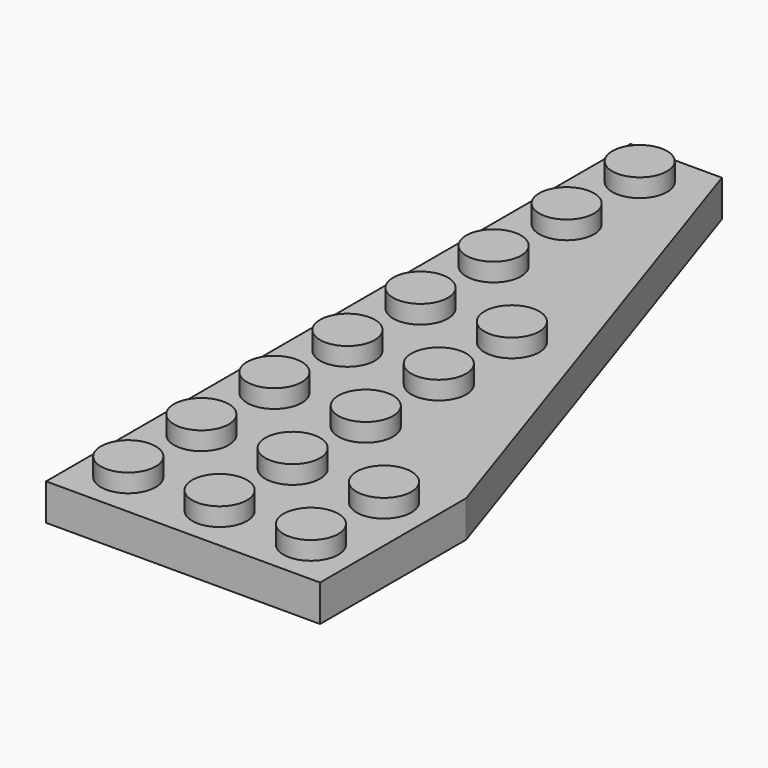
from build123d import *

# Parameters (mm, degrees)
F0_R     = 2.38125
F1_DEPTH = 3.175
F2_DEPTH = 4.7625
F3_T     = -1.5875
F4_R     = 3.175
F4_R_2   = 2.38125
F5_DEPTH = 1.5875


with BuildPart() as f1:
    # F0 (on Top) → F1 (new body)
    with BuildSketch(Plane.XY):
        Polygon((-3.96875, 31.75), (-11.90625, 31.75), (-11.90625, -31.75), (11.90625, -31.75), (11.90625, -15.875), align=None)
        with Locations((-7.9375, -27.78125)):
            Circle(F0_R, mode=Mode.SUBTRACT)
        with Locations((-7.9375, -19.84375)):
            Circle(F0_R, mode=Mode.SUBTRACT)
        with Locations((-7.9375, -11.90625)):
            Circle(F0_R, mode=Mode.SUBTRACT)
        with Locations((-7.9375, -3.96875)):
            Circle(F0_R, mode=Mode.SUBTRACT)
        with Locations((0, -27.78125)):
            Circle(F0_R, mode=Mode.SUBTRACT)
        with Locations((0, -19.84375)):
            Circle(F0_R, mode=Mode.SUBTRACT)
        with Locations((7.9375, -27.78125)):
            Circle(F0_R, mode=Mode.SUBTRACT)
        with Locations((7.9375, -19.84375)):
            Circle(F0_R, mode=Mode.SUBTRACT)
        with Locations((0, -11.90625)):
            Circle(F0_R, mode=Mode.SUBTRACT)
        with Locations((0, -3.96875)):
            Circle(F0_R, mode=Mode.SUBTRACT)
        with Locations((-7.9375, 3.96875)):
            Circle(F0_R, mode=Mode.SUBTRACT)
        with Locations((-7.9375, 11.90625)):
            Circle(F0_R, mode=Mode.SUBTRACT)
        with Locations((-7.9375, 19.84375)):
            Circle(F0_R, mode=Mode.SUBTRACT)
        with Locations((-7.9375, 27.78125)):
            Circle(F0_R, mode=Mode.SUBTRACT)
        with Locations((0, 3.96875)):
            Circle(F0_R, mode=Mode.SUBTRACT)
    extrude(amount=F1_DEPTH)

    # F0 (on Top) → F2 (join)
    with BuildSketch(Plane.XY):
        with Locations((-7.9375, 27.78125)):
            Circle(F0_R)
        with Locations((-7.9375, 19.84375)):
            Circle(F0_R)
        with Locations((-7.9375, 11.90625)):
            Circle(F0_R)
        with Locations((-7.9375, 3.96875)):
            Circle(F0_R)
        with Locations((-7.9375, -3.96875)):
            Circle(F0_R)
        with Locations((-7.9375, -11.90625)):
            Circle(F0_R)
        with Locations((-7.9375, -19.84375)):
            Circle(F0_R)
        with Locations((-7.9375, -27.78125)):
            Circle(F0_R)
        with Locations((0, -27.78125)):
            Circle(F0_R)
        with Locations((0, -19.84375)):
            Circle(F0_R)
        with Locations((0, -11.90625)):
            Circle(F0_R)
        with Locations((0, -3.96875)):
            Circle(F0_R)
        with Locations((0, 3.96875)):
            Circle(F0_R)
        with Locations((7.9375, -19.84375)):
            Circle(F0_R)
        with Locations((7.9375, -27.78125)):
            Circle(F0_R)
    extrude(amount=F2_DEPTH)

    # F3
    f3_openings = [f1.faces().sort_by_distance(p)[0] for p in [
        (-2.204861, -5.291667, 0),
    ]]
    offset(amount=F3_T, openings=f3_openings, kind=Kind.INTERSECTION)

    # F4 (on face) → F5 (join)
    with BuildSketch(Plane(origin=(0, 0, 1.5875), x_dir=(1, 0, 0), z_dir=(0, 0, -1))):
        with BuildLine():
            ThreePointArc((1.7236859697, 26.0575640303), (1.7236859697, 21.5674359697), (6.2138140303, 21.5674359697))
            Line((6.2138140303, 21.5674359697), (5.6525480227, 22.1287019773))
            ThreePointArc((5.6525480227, 22.1287019773), (2.2849519773, 22.1287019773), (2.2849519773, 25.4962980227))
            Line((2.2849519773, 25.4962980227), (1.7236859697, 26.0575640303))
        make_face()
        with BuildLine():
            Line((5.6525480227, 22.1287019773), (6.2138140303, 21.5674359697))
            ThreePointArc((6.2138140303, 21.5674359697), (6.9020675157, 22.5974801022), (7.14375, 23.8125))
            ThreePointArc((7.14375, 23.8125), (5.1837698978, 26.7458175157), (1.7236859697, 26.0575640303))
            Line((1.7236859697, 26.0575640303), (2.2849519773, 25.4962980227))
            ThreePointArc((2.2849519773, 25.4962980227), (4.8800149233, 26.0124881368), (6.35, 23.8125))
            ThreePointArc((6.35, 23.8125), (6.1687381368, 22.9012350767), (5.6525480227, 22.1287019773))
        make_face()
        with Locations((3.96875, 15.875)):
            Circle(F4_R)
        with Locations((3.96875, 15.875)):
            Circle(F4_R_2, mode=Mode.SUBTRACT)
        with Locations((3.96875, 7.9375)):
            Circle(F4_R)
        with Locations((3.96875, 7.9375)):
            Circle(F4_R_2, mode=Mode.SUBTRACT)
        with BuildLine():
            Line((5.5381726179, 1.7908836392), (5.8046687532, 2.590372045))
            ThreePointArc((5.8046687532, 2.590372045), (0.9566805287, 1.0040231571), (3.8832617755, -3.1738488879))
            Line((3.8832617755, -3.1738488879), (4.1497579108, -2.3743604821))
            ThreePointArc((4.1497579108, -2.3743604821), (1.7096978965, 0.7530173678), (5.5381726179, 1.7908836392))
        make_face()
        with BuildLine():
            Line((-2.3993273821, -22.0216163608), (-2.1328312468, -21.222127955))
            ThreePointArc((-2.1328312468, -21.222127955), (-6.9808194713, -22.8084768429), (-4.0542382245, -26.9863488879))
            Line((-4.0542382245, -26.9863488879), (-3.7877420892, -26.1868604821))
            ThreePointArc((-3.7877420892, -26.1868604821), (-6.2278021035, -23.0594826322), (-2.3993273821, -22.0216163608))
        make_face()
        with Locations((-3.96875, 23.8125)):
            Circle(F4_R)
        with Locations((-3.96875, 23.8125)):
            Circle(F4_R_2, mode=Mode.SUBTRACT)
        with Locations((-3.96875, 15.875)):
            Circle(F4_R)
        with Locations((-3.96875, 15.875)):
            Circle(F4_R_2, mode=Mode.SUBTRACT)
        with Locations((-3.96875, 7.9375)):
            Circle(F4_R)
        with Locations((-3.96875, 7.9375)):
            Circle(F4_R_2, mode=Mode.SUBTRACT)
        with Locations((-3.96875, 0)):
            Circle(F4_R)
        with Locations((-3.96875, 0)):
            Circle(F4_R_2, mode=Mode.SUBTRACT)
        with Locations((-3.96875, -7.9375)):
            Circle(F4_R)
        with Locations((-3.96875, -7.9375)):
            Circle(F4_R_2, mode=Mode.SUBTRACT)
        with Locations((-3.96875, -15.875)):
            Circle(F4_R)
        with Locations((-3.96875, -15.875)):
            Circle(F4_R_2, mode=Mode.SUBTRACT)
    extrude(amount=F5_DEPTH)


solid = f1.part
